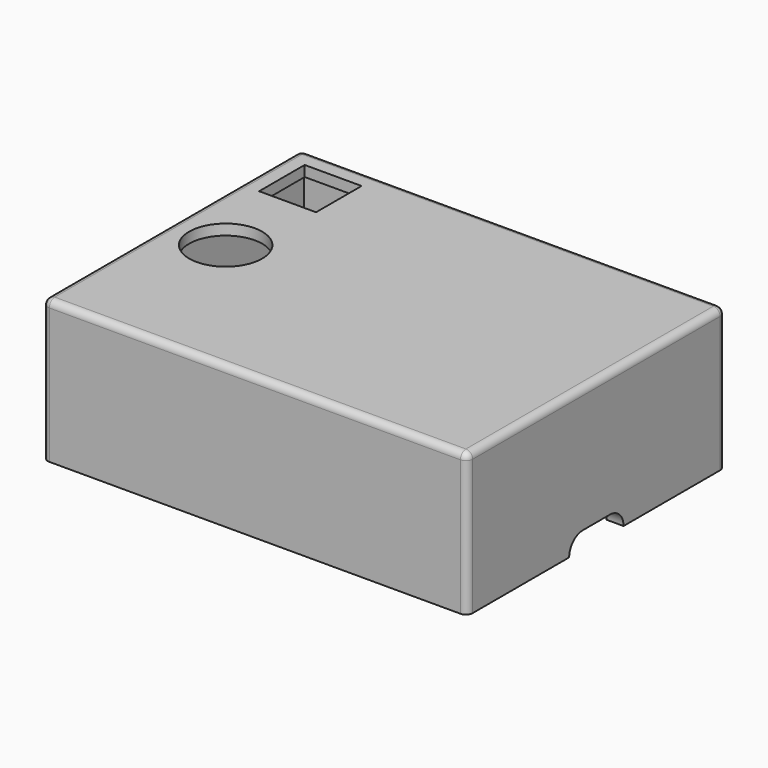
from build123d import *

# Parameters (mm, degrees)
F0_W     = 127
F0_H     = 96.52
F0_R     = 10.922
F0_W_2   = 17.018
F0_H_2   = 17.018
F1_DEPTH = 3.175
F2_W     = 127
F2_H     = 96.52
F2_W_2   = 116.8399999365
F2_H_2   = 86.3599999365
F3_DEPTH = 39.37
F4_R     = 2.032
F5_W     = 5.0800000317
F5_H     = 20.32
F6_DEPTH = 5.08
F7_R     = 5.07999


# Not quite as in the source:
# - a fillet or chamfer is up to 0.001 mm smaller than in the source, because OpenCascade refuses the exact size


with BuildPart() as f1:
    # F0 (on Top) → F1 (new body)
    with BuildSketch(Plane.XY):
        with Locations((63.5, 48.26)):
            Rectangle(F0_W, F0_H)
        with Locations((16.764, 47.498)):
            Circle(F0_R, mode=Mode.SUBTRACT)
        with Locations((14.351, 82.169)):
            Rectangle(F0_W_2, F0_H_2, mode=Mode.SUBTRACT)
    extrude(amount=F1_DEPTH)

    # F2 (on face) → F3 (join)
    with BuildSketch(Plane(origin=(0, 0, 0), x_dir=(1, 0, 0), z_dir=(0, 0, -1))):
        with Locations((63.5, -48.26)):
            Rectangle(F2_W, F2_H)
        with Locations((63.5, -48.26)):
            Rectangle(F2_W_2, F2_H_2, mode=Mode.SUBTRACT)
    extrude(amount=F3_DEPTH)

    # F4
    f4_edges = [f1.edges().sort_by_distance(p)[0] for p in [
        (0, 96.52, -18.0975),
        (63.5, 96.52, 3.175),
        (0, 48.26, 3.175),
        (127, 96.52, -18.0975),
        (127, 48.26, 3.175),
        (127, 0, -18.0975),
        (63.5, 0, 3.175),
        (0, 0, -18.0975),
    ]]
    fillet(f4_edges, radius=F4_R)

    # F5 (on face) → F6 (cut)
    with BuildSketch(Plane(origin=(0, 0, -39.37), x_dir=(1, 0, 0), z_dir=(0, 0, -1))):
        with Locations((124.4599999841, -48.26)):
            Rectangle(F5_W, F5_H)
        with Locations((2.5400000159, -48.26)):
            Rectangle(F5_W, F5_H)
    extrude(amount=-F6_DEPTH, mode=Mode.SUBTRACT)

    # F7 (radius 5.08 in the source; OpenCascade refuses exactly that, so slightly less here)
    f7_edges = [f1.edges().sort_by_distance(p)[0] for p in [
        (2.54, 38.1, -34.29),
        (2.54, 58.42, -34.29),
        (124.46, 58.42, -34.29),
        (124.46, 38.1, -34.29),
    ]]
    fillet(f7_edges, radius=F7_R)


solid = f1.part
